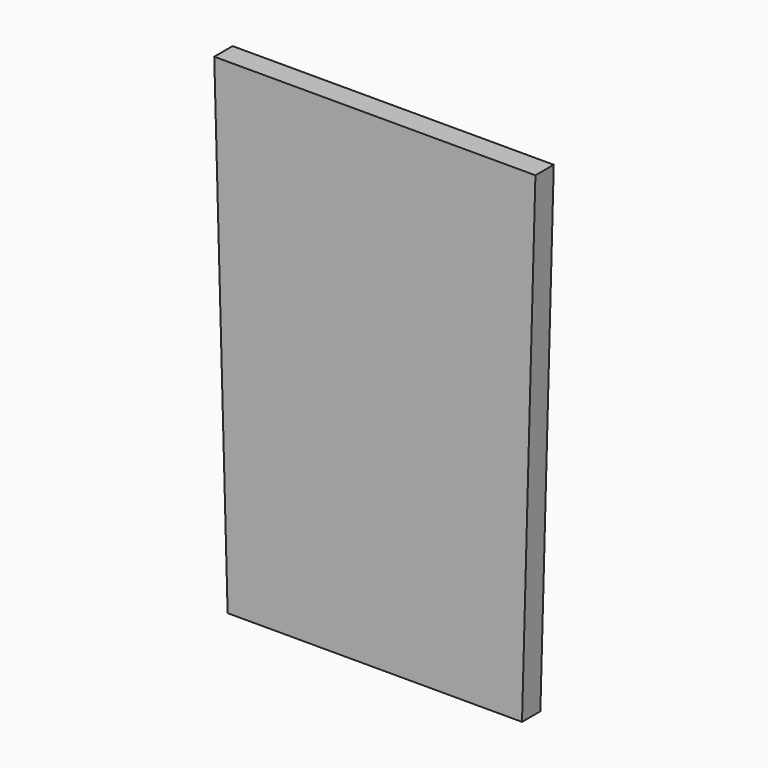
from build123d import *

# Parameters (mm, degrees)
F1_DEPTH = 19.05


# Not quite as in the source:
# - a length typed as a fraction of an inch, garbled in the dataset ("3 / 203.2 mm" for 3/8 in), is restored


with BuildPart() as f1:
    # F0 (on Front) → F1 (new body)
    with BuildSketch(Plane.XZ):
        Polygon((133.35, 0), (0, 0), (-133.35, 0), (-122.2375, -403.225), (0, -403.225), (122.2375, -403.225), align=None)
    extrude(amount=F1_DEPTH)


solid = f1.part
